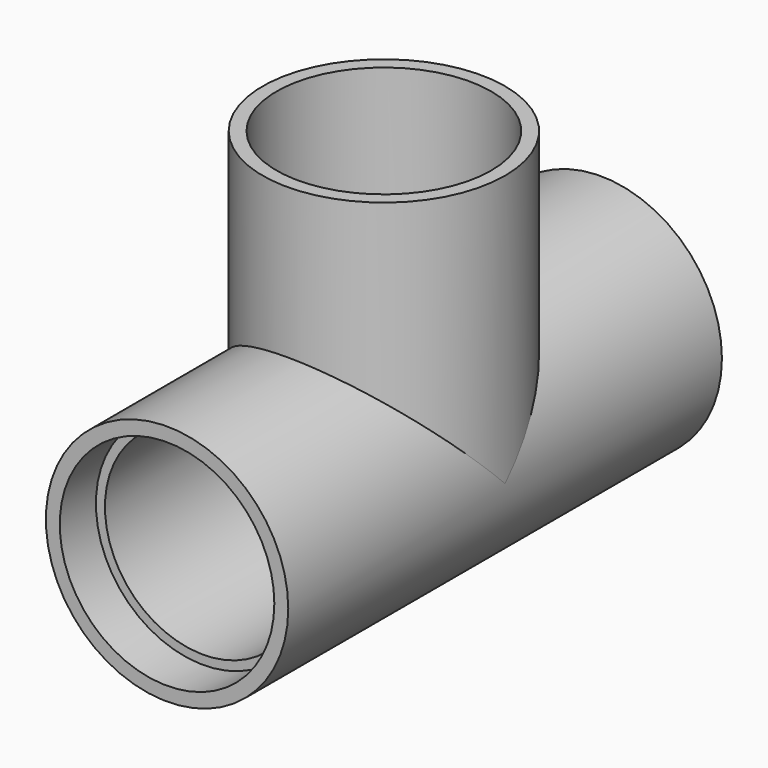
from build123d import *
from build123d import SkipClean  # not in build123d's __all__

# Parameters (mm, degrees)
F0_R     = 34.0741
F0_R_2   = 30.1625
F1_DEPTH = 76.2
F2_R     = 34.0741
F2_R_2   = 30.1625
F3_DEPTH = 76.2
F4_R     = 34.0741
F4_R_2   = 27.6225
F5_DEPTH = 63.5
F6_R     = 30.1625
F7_DEPTH = 76.2
F8_R     = 27.6225
F9_DEPTH = 143.6


with BuildPart() as f1:
    # F0 (on Front) → F1 (new body, symmetric)
    with BuildSketch(Plane.XZ):
        Circle(F0_R)
        Circle(F0_R_2, mode=Mode.SUBTRACT)
    extrude(amount=F1_DEPTH, both=True)

    # F2 (on Top) → F3 (join)
    with BuildSketch(Plane.XY):
        Circle(F2_R)
        Circle(F2_R_2, mode=Mode.SUBTRACT)
    extrude(amount=F3_DEPTH)

    # F4 (on Front) → F5 (join, symmetric)
    with BuildSketch(Plane.XZ):
        Circle(F4_R)
        Circle(F4_R_2, mode=Mode.SUBTRACT)
    with SkipClean():  # cleaning this boolean's faces spoils the solid; the shape is the same uncleaned
        extrude(amount=F5_DEPTH, both=True)

    # F6 (on face) → F7 (cut, through all)
    with BuildSketch(Plane.XY.offset(76.2)):
        Circle(F6_R)
    extrude(amount=-F7_DEPTH, mode=Mode.SUBTRACT)

    # F8 (on Front) → F9 (cut, symmetric)
    with BuildSketch(Plane.XZ):
        Circle(F8_R)
    extrude(amount=F9_DEPTH, both=True, mode=Mode.SUBTRACT)


solid = f1.part
